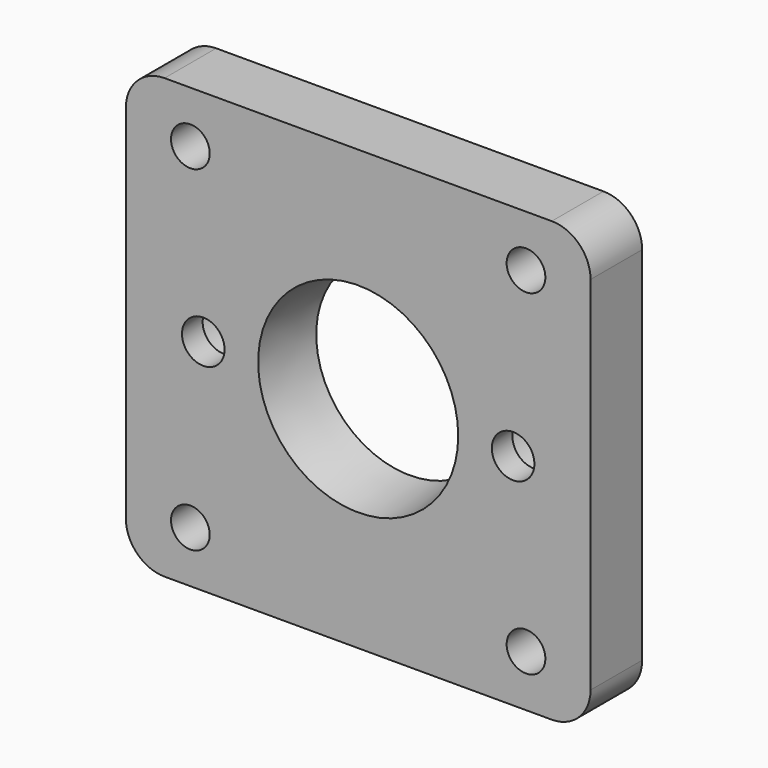
from build123d import *

# Parameters (mm, degrees)
F0_W           = 36
F0_H           = 34
F0_R           = 1.5
F0_R_2         = 7.25
F1_DEPTH       = 5
F2_R           = 3
F3_SIZE2       = 4.99999
F3_SIZE        = 0.49999
F4_D           = 3.3
F4_CBORE_D     = 6.5
F4_CBORE_DEPTH = 3


# Not quite as in the source:
# - a fillet or chamfer is up to 0.001 mm smaller than in the source, because OpenCascade refuses the exact size


with BuildPart() as f1:
    # F0 (on Front) → F1 (new body)
    with BuildSketch(Plane.XZ):
        Rectangle(F0_W, F0_H)
        with Locations((-13, -13)):
            Circle(F0_R, mode=Mode.SUBTRACT)
        with Locations((13, -13)):
            Circle(F0_R, mode=Mode.SUBTRACT)
        with Locations((-13, 13)):
            Circle(F0_R, mode=Mode.SUBTRACT)
        Circle(F0_R_2, mode=Mode.SUBTRACT)
        with Locations((13, 13)):
            Circle(F0_R, mode=Mode.SUBTRACT)
    extrude(amount=F1_DEPTH)

    # F2
    f2_edges = [f1.edges().sort_by_distance(p)[0] for p in [
        (-18, -2.5, 17),
        (18, -2.5, 17),
        (18, -2.5, -17),
        (-18, -2.5, -17),
    ]]
    fillet(f2_edges, radius=F2_R)

    # F3 (size 0.5 and 5 in the source; OpenCascade refuses exactly that, so slightly less here)
    f3_edges = [f1.edges().sort_by_distance(p)[0] for p in [
        (-7.25, -5, 0),
    ]]
    f3_side = f1.faces().sort_by_distance((0, -5, -16.504823))[0]
    chamfer(f3_edges, length=F3_SIZE, length2=F3_SIZE2, reference=f3_side)

    # F4 (through all)
    with Locations(Plane(origin=(0, 0, 0), x_dir=(1, 0, 0), z_dir=(0, 1, 0))):
        with Locations((12, 0), (-12, 0)):
            CounterBoreHole(F4_D / 2, F4_CBORE_D / 2, F4_CBORE_DEPTH)


solid = f1.part
